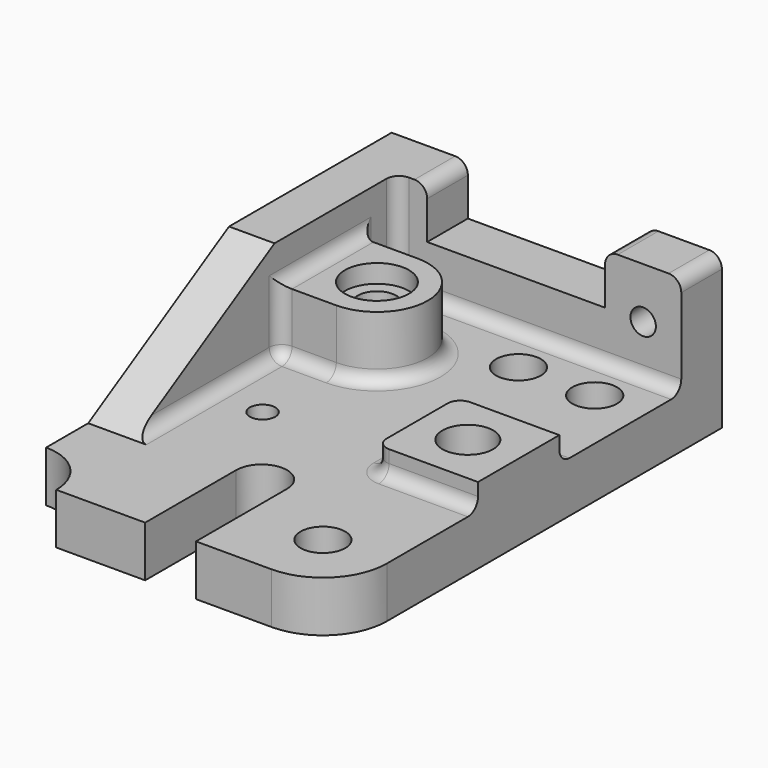
from build123d import *

# Parameters (mm, degrees)
F0_W      = 82.55
F0_H      = 120.65
F1_DEPTH  = 12.7
F3_DEPTH  = 25.4
F5_DEPTH  = 11.3716514647
F6_W      = 44.45
F6_H      = 12.7
F7_DEPTH  = 25.4
F8_W      = 25.4
F8_H      = 25.4
F9_DEPTH  = 6.35
F10_R     = 6.35
F11_DEPTH = 19.051
F13_DEPTH = 15.748
F14_R     = 4.826
F15_DEPTH = 28.449
F16_R     = 8.001
F16_R_2   = 4.826
F17_DEPTH = 4.572
F18_W     = 12.7
F18_H     = 28.448
F19_DEPTH = 25.4
F20_R     = 3.175
F20_R_2   = 5.588
F21_DEPTH = 12.701
F22_R     = 3.175
F23_DEPTH = 25.4
F25_DEPTH = 25.4
F26_R     = 16.002
F27_R     = 3.175


with BuildPart() as f1:
    # F0 (on Top) → F1 (new body)
    with BuildSketch(Plane.XY):
        with Locations((-0.8694417775, 29.0160470424)):
            Rectangle(F0_W, F0_H)
    extrude(amount=F1_DEPTH)

    # F2 (on face) → F3 (join)
    with BuildSketch(Plane.XY.offset(12.7)):
        Polygon((-30.7727903128, 89.3410470424), (-42.1444417775, 89.3410470424), (-42.1444417775, 76.6410470424), (-42.1444417775, 38.5410470424), (-30.7727903128, 38.5410470424), (-30.7727903128, 76.6410470424), (40.4055582225, 76.6410470424), (40.4055582225, 89.3410470424), align=None)
    extrude(amount=F3_DEPTH)

    # F4 (on face) → F5 (join, through all)
    with BuildSketch(Plane.YZ.offset(-30.7727903128)):
        Polygon((38.5410470424, 12.7), (38.5410470424, 38.1), (-5.4530434699, 12.7), align=None)
    extrude(amount=-F5_DEPTH)

    # F6 (on face) → F7 (cut)
    with BuildSketch(Plane(origin=(0, 89.3410470424, 0), x_dir=(-1, 0, 0), z_dir=(0, 1, 0))):
        with Locations((0.8694417775, 31.75)):
            Rectangle(F6_W, F6_H)
    extrude(amount=-F7_DEPTH, mode=Mode.SUBTRACT)

    # F8 (on face) → F9 (join)
    with BuildSketch(Plane.XY.offset(12.7)):
        with Locations((27.7055582225, 25.8410470424)):
            Rectangle(F8_W, F8_H)
    extrude(amount=F9_DEPTH)

    # F10 (on face) → F11 (cut, through all)
    with BuildSketch(Plane.XY.offset(19.05)):
        with Locations((27.7055582225, 25.8410470424)):
            Circle(F10_R)
    extrude(amount=-F11_DEPTH, mode=Mode.SUBTRACT)

    # F12 (on face) → F13 (join)
    with BuildSketch(Plane.XY.offset(12.7)):
        with BuildLine():
            Line((-30.7727903128, 65.4650470424), (-30.7727903128, 40.0650470424))
            Line((-30.7727903128, 40.0650470424), (-16.5487903128, 40.0650470424))
            ThreePointArc((-16.5487903128, 40.0650470424), (-3.8487903128, 52.7650470424), (-16.5487903128, 65.4650470424))
            Line((-16.5487903128, 65.4650470424), (-30.7727903128, 65.4650470424))
        make_face()
    extrude(amount=F13_DEPTH)

    # F14 (on face) → F15 (cut, through all)
    with BuildSketch(Plane.XY.offset(28.448)):
        with Locations((-16.5487903128, 52.7650470424)):
            Circle(F14_R)
    extrude(amount=-F15_DEPTH, mode=Mode.SUBTRACT)

    # F16 (on face) → F17 (cut)
    with BuildSketch(Plane.XY.offset(28.448)):
        with Locations((-16.5487903128, 52.7650470424)):
            Circle(F16_R)
        with Locations((-16.5487903128, 52.7650470424)):
            Circle(F16_R_2, mode=Mode.SUBTRACT)
    extrude(amount=-F17_DEPTH, mode=Mode.SUBTRACT)

    # F18 (on face) → F19 (cut)
    with BuildSketch(Plane.XY.offset(12.7)):
        with Locations((-0.8694417775, -17.0849529576)):
            Rectangle(F18_W, F18_H)
        with BuildLine():
            ThreePointArc((5.4805582225, -2.8609529576), (-0.8694417775, 3.4890470424), (-7.2194417775, -2.8609529576))
            Line((-7.2194417775, -2.8609529576), (5.4805582225, -2.8609529576))
        make_face()
    extrude(amount=-F19_DEPTH, mode=Mode.SUBTRACT)

    # F20 (on face) → F21 (cut, through all)
    with BuildSketch(Plane.XY.offset(12.7)):
        with Locations((-18.5224417775, 19.4910470424)):
            Circle(F20_R)
        with Locations((24.4035582225, -15.3069529576)):
            Circle(F20_R_2)
        with Locations((27.7055582225, 65.4650470424)):
            Circle(F20_R_2)
        with Locations((8.6555582225, 65.4650470424)):
            Circle(F20_R_2)
    extrude(amount=-F21_DEPTH, mode=Mode.SUBTRACT)

    # F22 (on face) → F23 (cut)
    with BuildSketch(Plane.XZ.offset(-76.6410470424)):
        with Locations((30.8805582225, 25.4)):
            Circle(F22_R)
    extrude(amount=-F23_DEPTH, mode=Mode.SUBTRACT)

    # F24 (on face) → F25 (cut)
    with BuildSketch(Plane.XY.offset(12.7)):
        with BuildLine():
            Line((-42.1444417775, -31.3089529576), (-29.4444417775, -31.3089529576))
            ThreePointArc((-29.4444417775, -31.3089529576), (-33.1641856564, -22.3286968366), (-42.1444417775, -18.6089529576))
            Line((-42.1444417775, -18.6089529576), (-42.1444417775, -31.3089529576))
        make_face()
    extrude(amount=-F25_DEPTH, mode=Mode.SUBTRACT)

    # F26
    f26_edges = [f1.edges().sort_by_distance(p)[0] for p in [
        (40.405558, -31.308953, 6.35),
    ]]
    fillet(f26_edges, radius=F26_R)

    # F27
    f27_edges = [f1.edges().sort_by_distance(p)[0] for p in [
        (-30.77279, 17.306002, 12.7),
        (-30.77279, 40.065047, 20.574),
        (-23.66079, 40.065047, 12.7),
        (-30.77279, 52.765047, 28.448),
        (4.816384, 76.641047, 12.7),
        (-30.77279, 65.465047, 20.574),
        (-30.77279, 76.641047, 25.4),
        (15.005558, 13.141047, 15.875),
        (15.005558, 38.541047, 15.875),
        (-23.094442, 82.991047, 38.1),
        (40.405558, 82.991047, 38.1),
        (21.355558, 82.991047, 38.1),
        (27.705558, 13.141047, 12.7),
        (15.005558, 25.841047, 12.7),
        (27.705558, 38.541047, 12.7),
        (-23.66079, 65.465047, 12.7),
        (-3.84879, 52.765047, 12.7),
    ]]
    fillet(f27_edges, radius=F27_R)


solid = f1.part
